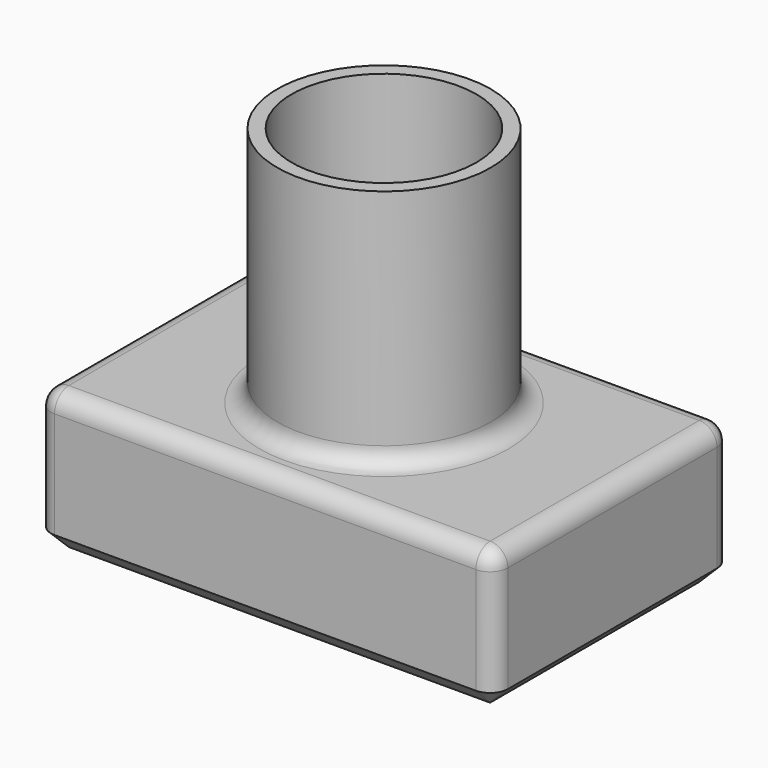
from build123d import *

# Parameters (mm, degrees)
F0_W     = 12.85
F0_H     = 8.35
F1_DEPTH = 4
F2_R     = 3
F3_DEPTH = 6.8
F4_R     = 2.6
F5_DEPTH = 10.801
F6_R     = 0.5
F7_R     = 0.5
F8_SIZE  = 0.49999


# Not quite as in the source:
# - a fillet or chamfer is up to 0.001 mm smaller than in the source, because OpenCascade refuses the exact size


with BuildPart() as f1:
    # F0 (on Top) → F1 (new body)
    with BuildSketch(Plane.XY):
        Rectangle(F0_W, F0_H)
    extrude(amount=F1_DEPTH)

    # F2 (on face) → F3 (join)
    with BuildSketch(Plane.XY.offset(4)):
        Circle(F2_R)
    extrude(amount=F3_DEPTH)

    # F4 (on face) → F5 (cut, through all)
    with BuildSketch(Plane.XY.offset(10.8)):
        Circle(F4_R)
    extrude(amount=-F5_DEPTH, mode=Mode.SUBTRACT)

    # F6
    f6_edges = [f1.edges().sort_by_distance(p)[0] for p in [
        (-6.425, 4.175, 2),
        (6.425, 4.175, 2),
        (6.425, -4.175, 2),
        (-6.425, -4.175, 2),
    ]]
    fillet(f6_edges, radius=F6_R)

    # F7
    f7_edges = [f1.edges().sort_by_distance(p)[0] for p in [
        (0, -4.175, 4),
        (-6.278553, -4.028553, 4),
        (6.278553, -4.028553, 4),
        (-6.425, 0, 4),
        (6.425, 0, 4),
        (-6.278553, 4.028553, 4),
        (6.278553, 4.028553, 4),
        (0, 4.175, 4),
        (-3, 0, 4),
    ]]
    fillet(f7_edges, radius=F7_R)

    # F8 (size 0.5 in the source; OpenCascade refuses exactly that, so slightly less here)
    f8_edges = [f1.edges().sort_by_distance(p)[0] for p in [
        (0, -4.175, 0),
        (-6.278553, -4.028553, 0),
        (6.278553, -4.028553, 0),
        (-6.425, 0, 0),
        (6.425, 0, 0),
        (-6.278553, 4.028553, 0),
        (6.278553, 4.028553, 0),
        (0, 4.175, 0),
        (-2.6, 0, 0),
    ]]
    chamfer(f8_edges, length=F8_SIZE)


solid = f1.part
